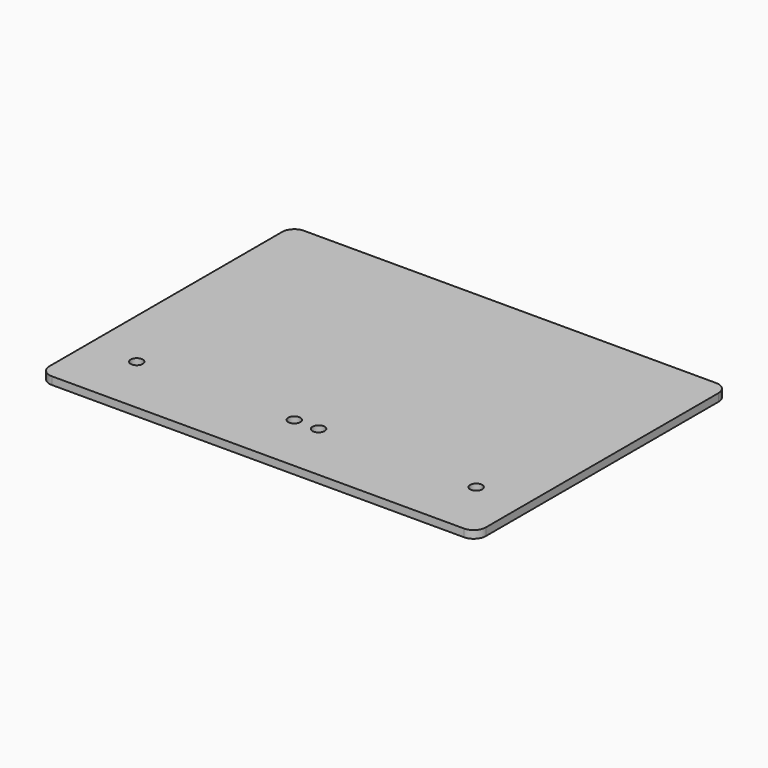
from build123d import *

# Parameters (mm, degrees)
F0_W     = 180
F0_H     = 130
F0_R     = 2.5
F1_DEPTH = 1.5875
F2_R     = 5


# Not quite as in the source:
# - a length typed as a fraction of an inch, garbled in the dataset ("3 / 203.2 mm" for 3/8 in), is restored


with BuildPart() as f1:
    # F0 (on Top) → F1 (new body, symmetric)
    with BuildSketch(Plane.XY):
        Rectangle(F0_W, F0_H)
        with Locations((-70, -40)):
            Circle(F0_R, mode=Mode.SUBTRACT)
        with Locations((-5, -40)):
            Circle(F0_R, mode=Mode.SUBTRACT)
        with Locations((5, -40)):
            Circle(F0_R, mode=Mode.SUBTRACT)
        with Locations((70, -40)):
            Circle(F0_R, mode=Mode.SUBTRACT)
    extrude(amount=F1_DEPTH, both=True)

    # F2
    f2_edges = [f1.edges().sort_by_distance(p)[0] for p in [
        (-90, 65, 0),
        (-90, -65, 0),
        (90, -65, 0),
        (90, 65, 0),
    ]]
    fillet(f2_edges, radius=F2_R)


solid = f1.part
